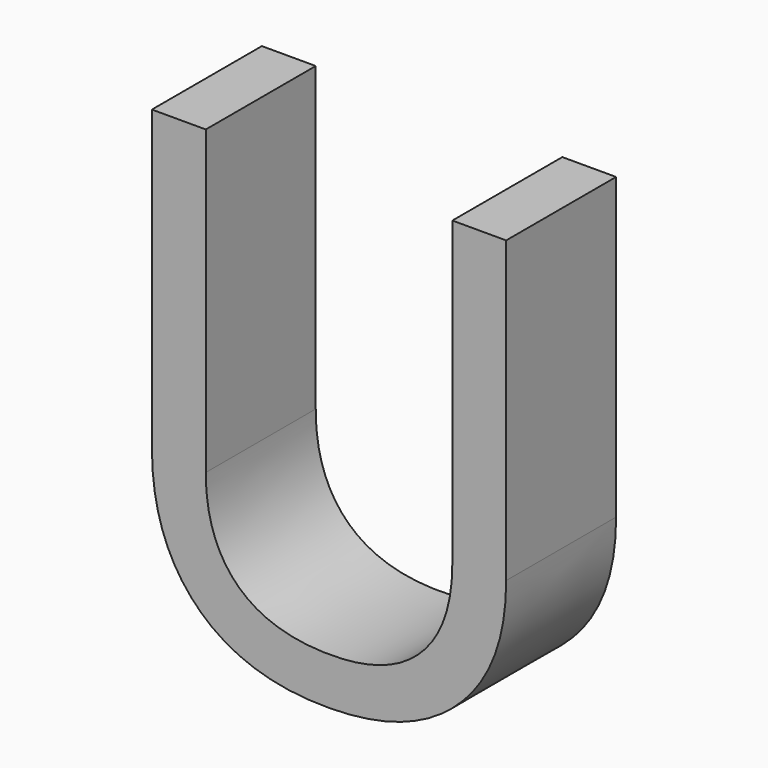
from build123d import *

# Parameters (mm, degrees)
F0_TEXT_SIZE = 47.1721920702
F1_DEPTH     = 10


# Not quite as in the source:
# - Text() gives the source's letters only with a copy of the font that has no kerning and outlines rounded to 1/6400 em; it was checked with that copy


with BuildPart() as f1:
    # F0 (on Front) → F1 (new body)
    with BuildSketch(Plane.XZ):
        with Locations((-33.1163529643, 0)):
            Text('U', F0_TEXT_SIZE, font='Open Sans', text_align=(TextAlign.LEFT, TextAlign.BOTTOM))
    extrude(amount=F1_DEPTH)


solid = f1.part
